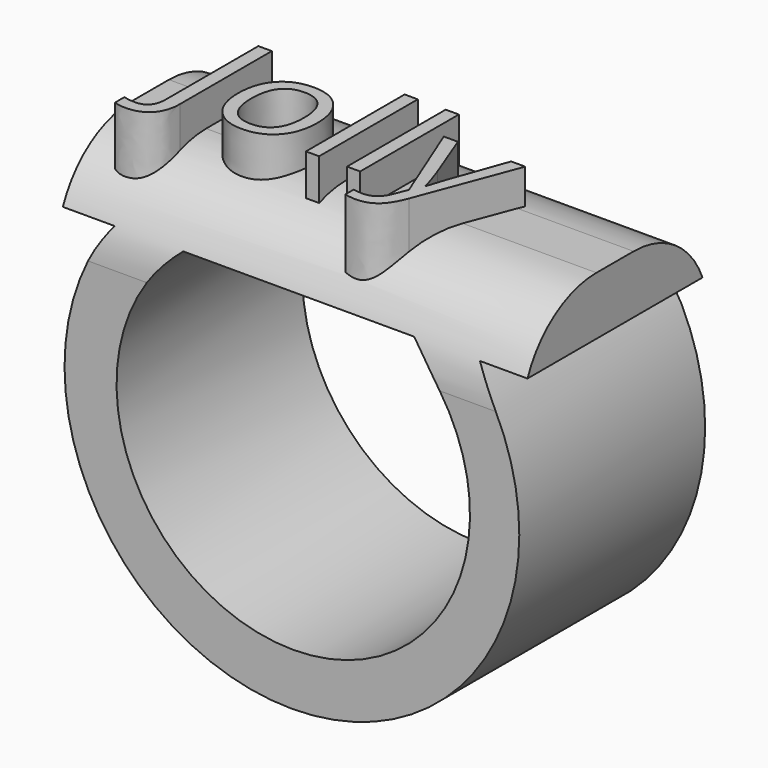
from build123d import *

# Parameters (mm, degrees)
F0_W         = 25.4
F0_H         = 12.7
F1_DEPTH     = 3.175
F3_DEPTH     = 12.7
F5_T1_DEPTH  = 50.8
F4_TEXT_SIZE = 8.8730348378
F6_DEPTH     = 5.08


# Not quite as in the source:
# - a fillet or chamfer that OpenCascade refuses, or shapes differently, is made with other operations: its cross-section is extruded or revolved along the edge and cut away or added
# - Text() gives the source's letters only with a copy of the font that has no kerning and outlines rounded to 1/6400 em; it was checked with that copy


with BuildPart() as f1:
    # F0 (on Top) → F1 (new body)
    with BuildSketch(Plane.XY):
        with Locations((-0.7055559625, -6.35)):
            Rectangle(F0_W, F0_H)
    extrude(amount=F1_DEPTH)

    # F2 (on Front) → F3 (join)
    with BuildSketch(Plane.XZ):
        with BuildLine():
            Line((-6.8265399896, 0), (-10.570127517, 0))
            ThreePointArc((-10.570127517, 0), (-0.58722822, -19.8342574736), (9.3956710771, 0))
            Line((9.3956710771, 0), (5.7988902554, 0))
            ThreePointArc((5.7988902554, 0), (-0.5138248671, -16.9728395932), (-6.8265399896, 0))
        make_face()
    extrude(amount=F3_DEPTH)

    # F5: fillet of radius 5.08 on 2 edges, made by hand

    # F5_s2 → F5_t1 (cut)
    with BuildSketch(Plane.YZ.offset(-26.1055559625)):
        with BuildLine():
            ThreePointArc((0, -1.905), (-1.4878975516, 1.6871024484), (-5.08, 3.175))
            Line((-5.08, 3.175), (0, 3.175))
            Line((0, 3.175), (0, -1.905))
        make_face()
        with BuildLine():
            ThreePointArc((-12.7, -1.905), (-11.2121024484, 1.6871024484), (-7.62, 3.175))
            Line((-7.62, 3.175), (-12.7, 3.175))
            Line((-12.7, 3.175), (-12.7, -1.905))
        make_face()
    extrude(amount=F5_T1_DEPTH, mode=Mode.SUBTRACT)

    # F4 (on Top) → F6 (join)
    with BuildSketch(Plane.XY):
        with Locations((-10.9029849991, -9.4615900889)):
            Text('Jolly', F4_TEXT_SIZE, font='Open Sans', text_align=(TextAlign.LEFT, TextAlign.BOTTOM))
    extrude(amount=F6_DEPTH)


solid = f1.part
